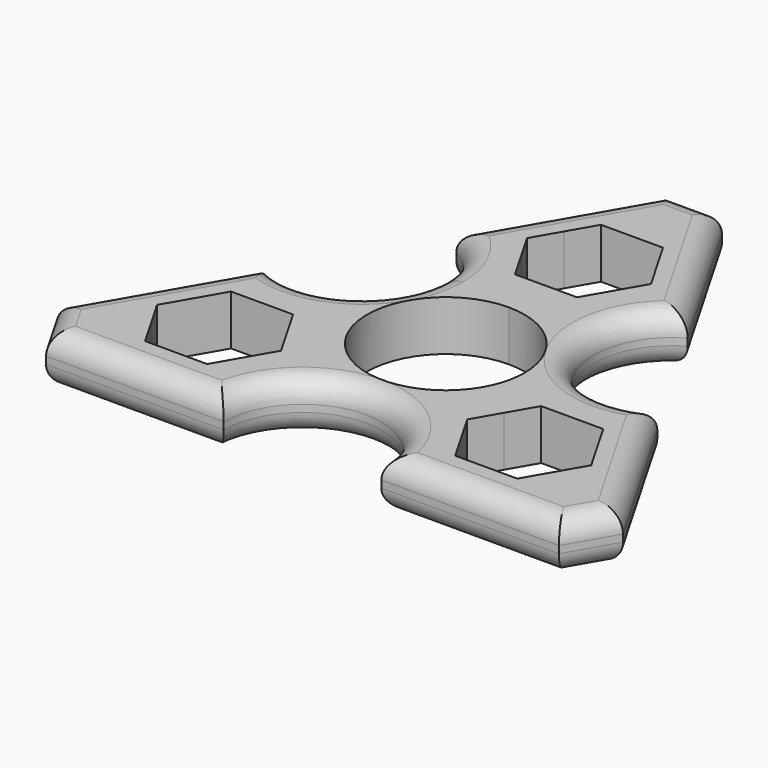
from build123d import *

# Parameters (mm, degrees)
F1_DEPTH      = 3.5
F1_DEPTH_BACK = 3.5
F2_SIZE       = 7.5
F3_R          = 2.99999
F4_R          = 2.99999


# Not quite as in the source:
# - a fillet or chamfer is up to 0.001 mm smaller than in the source, because OpenCascade refuses the exact size


with BuildPart() as f1:
    # F0 (on Top) → F1 (new body, two sides)
    with BuildSketch(Plane.XY) as f1_sk:
        with BuildLine():
            ThreePointArc((-9.526279, -5.5), (-9.526279, 5.5), (0, 11))
            Line((0, 11), (0, 17.5))
            Line((0, 17.5), (-4.330127, 17.5))
            Line((-4.330127, 17.5), (-6.495191, 21.25))
            Line((-6.495191, 21.25), (-8.660254, 25))
            Line((-8.660254, 25), (-6.495191, 28.75))
            Line((-6.495191, 28.75), (-4.330127, 32.5))
            Line((-4.330127, 32.5), (0, 32.5))
            Line((0, 32.5), (0, 50))
            Line((0, 50), (-16.150635, 22.026279))
            ThreePointArc((-16.150635, 22.026279), (-12.124356, 18), (-10.650635, 12.5))
            ThreePointArc((-10.650635, 12.5), (-16.150635, 2.973721), (-27.150635, 2.973721))
            Line((-27.150635, 2.973721), (-43.30127, -25))
            Line((-43.30127, -25), (-28.145826, -16.25))
            Line((-28.145826, -16.25), (-30.310889, -12.5))
            Line((-30.310889, -12.5), (-25.980762, -5))
            Line((-25.980762, -5), (-17.320508, -5))
            Line((-17.320508, -5), (-15.155445, -8.75))
            Line((-15.155445, -8.75), (-9.526279, -5.5))
        make_face()
        with BuildLine():
            ThreePointArc((0, 11), (7.778175, 7.778175), (11, 0))
            ThreePointArc((11, 0), (10.625184, -2.847009), (9.526279, -5.5))
            Line((9.526279, -5.5), (15.155445, -8.75))
            Line((15.155445, -8.75), (17.320508, -5))
            Line((17.320508, -5), (25.980762, -5))
            Line((25.980762, -5), (30.310889, -12.5))
            Line((30.310889, -12.5), (28.145826, -16.25))
            Line((28.145826, -16.25), (43.30127, -25))
            Line((43.30127, -25), (27.150635, 2.973721))
            ThreePointArc((27.150635, 2.973721), (12.124356, 7), (16.150635, 22.026279))
            Line((16.150635, 22.026279), (0, 50))
            Line((0, 50), (0, 32.5))
            Line((0, 32.5), (4.330127, 32.5))
            Line((4.330127, 32.5), (6.495191, 28.75))
            Line((6.495191, 28.75), (8.660254, 25))
            Line((8.660254, 25), (6.49519, 21.25))
            Line((6.49519, 21.25), (4.330127, 17.5))
            Line((4.330127, 17.5), (0, 17.5))
            Line((0, 17.5), (0, 11))
        make_face()
        with BuildLine():
            Line((15.155445, -8.75), (9.526279, -5.5))
            ThreePointArc((9.526279, -5.5), (0, -11), (-9.526279, -5.5))
            Line((-9.526279, -5.5), (-15.155445, -8.75))
            Line((-15.155445, -8.75), (-12.990381, -12.5))
            Line((-12.990381, -12.5), (-17.320508, -20))
            Line((-17.320508, -20), (-25.980762, -20))
            Line((-25.980762, -20), (-28.145826, -16.25))
            Line((-28.145826, -16.25), (-43.30127, -25))
            Line((-43.30127, -25), (-11, -25))
            ThreePointArc((-11, -25), (0, -14), (11, -25))
            Line((11, -25), (43.30127, -25))
            Line((43.30127, -25), (28.145826, -16.25))
            Line((28.145826, -16.25), (25.980762, -20))
            Line((25.980762, -20), (17.320508, -20))
            Line((17.320508, -20), (12.990381, -12.5))
            Line((12.990381, -12.5), (15.155445, -8.75))
        make_face()
    extrude(amount=F1_DEPTH)
    extrude(f1_sk.sketch, amount=-F1_DEPTH_BACK)

    # F2
    f2_edges = [f1.edges().sort_by_distance(p)[0] for p in [
        (0, 50, 0),
        (43.30127, -25, 0),
        (-43.30127, -25, 0),
    ]]
    chamfer(f2_edges, length=F2_SIZE)

    # F3 (radius 3 in the source; OpenCascade refuses exactly that, so slightly less here)
    f3_edges = [f1.edges().sort_by_distance(p)[0] for p in [
        (9.950318, 32.765544, 3.5),
        (12.124356, 7, 3.5),
        (33.350953, -7.765544, 3.5),
        (37.67627, -21.752405, 3.5),
        (23.400635, -25, 3.5),
        (0, -14, 3.5),
        (-23.400635, -25, 3.5),
        (-37.67627, -21.752405, 3.5),
        (-33.350953, -7.765544, 3.5),
        (-12.124356, 7, 3.5),
        (-9.950318, 32.765544, 3.5),
        (0, 43.504809, 3.5),
    ]]
    fillet(f3_edges, radius=F3_R)

    # F4 (radius 3 in the source; OpenCascade refuses exactly that, so slightly less here)
    f4_edges = [f1.edges().sort_by_distance(p)[0] for p in [
        (-37.67627, -21.752405, -3.5),
        (37.67627, -21.752405, -3.5),
        (0, 43.504809, -3.5),
        (-9.950318, 32.765544, -3.5),
        (-12.124356, 7, -3.5),
        (-33.350953, -7.765544, -3.5),
        (-23.400635, -25, -3.5),
        (0, -14, -3.5),
        (23.400635, -25, -3.5),
        (33.350953, -7.765544, -3.5),
        (12.124356, 7, -3.5),
        (9.950318, 32.765544, -3.5),
    ]]
    fillet(f4_edges, radius=F4_R)


solid = f1.part
